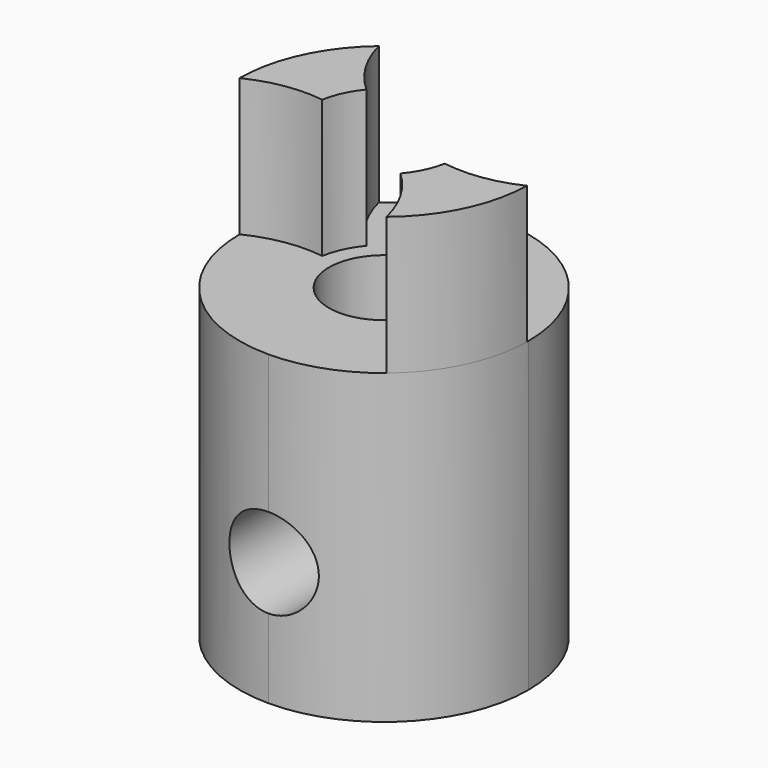
from build123d import *

# Parameters (mm, degrees)
F0_R        = 8.001
F0_R_2      = 3.048
F1_DEPTH    = 17.018
F3_W        = 16.002
F3_H        = 16.002
F4_DEPTH    = 17.018
F5_R        = 2.4765
F6_DEPTH    = 25.4
F7_T1_DEPTH = 57.023
F2_R        = 3.048
F8_DEPTH    = 25.4
F10_DEPTH   = 7.62
F11_SIZE    = 1.905


# Not quite as in the source:
# - a fillet or chamfer that OpenCascade refuses, or shapes differently, is made with other operations: its cross-section is extruded or revolved along the edge and cut away or added


with BuildPart() as f1:
    # F0 (on Top) → F1 (new body)
    with BuildSketch(Plane.XY):
        Circle(F0_R)
        Circle(F0_R_2, mode=Mode.SUBTRACT)
    extrude(amount=F1_DEPTH)

    # F3 (on Top) → F4 (join)
    with BuildSketch(Plane.XY):
        Rectangle(F3_W, F3_H)
    extrude(amount=F4_DEPTH)

    # F5 (on face) → F6 (cut)
    with BuildSketch(Plane.XZ.offset(8.001)):
        with Locations((0, 6.858)):
            Circle(F5_R)
    extrude(amount=-F6_DEPTH, mode=Mode.SUBTRACT)

    # F7: fillet of radius 8.001 on 4 edges, made by hand

    # F7_s2 → F7_t1 (cut)
    with BuildSketch(Plane.XY.offset(-20.0025)):
        with BuildLine():
            ThreePointArc((8.001, 0), (5.6575613563, -5.6575613563), (0, -8.001))
            Line((0, -8.001), (8.001, -8.001))
            Line((8.001, -8.001), (8.001, 0))
        make_face()
        with BuildLine():
            ThreePointArc((8.001, 0), (5.6575613563, 5.6575613563), (0, 8.001))
            Line((0, 8.001), (8.001, 8.001))
            Line((8.001, 8.001), (8.001, 0))
        make_face()
        with BuildLine():
            ThreePointArc((-8.001, 0), (-5.6575613563, -5.6575613563), (0, -8.001))
            Line((0, -8.001), (-8.001, -8.001))
            Line((-8.001, -8.001), (-8.001, 0))
        make_face()
        with BuildLine():
            ThreePointArc((0, 8.001), (-5.6575613563, 5.6575613563), (-8.001, 0))
            Line((-8.001, 0), (-8.001, 8.001))
            Line((-8.001, 8.001), (0, 8.001))
        make_face()
    extrude(amount=F7_T1_DEPTH, mode=Mode.SUBTRACT)

    # F2 (on face) → F8 (cut)
    with BuildSketch(Plane.XY.offset(17.018)):
        Circle(F2_R)
    extrude(amount=-F8_DEPTH, mode=Mode.SUBTRACT)

    # F9 (on face) → F10 (join)
    with BuildSketch(Plane.XY.offset(17.018)):
        with BuildLine():
            ThreePointArc((-3.0492599206, 2.589597302), (-4.3737921452, 4.1887242953), (-5.1697063492, 6.1065650953))
            ThreePointArc((-5.1697063492, 6.1065650953), (-7.2587471887, 3.3655), (-8.001, 0))
            ThreePointArc((-8.001, 0), (-6.0229894511, 0.6317175182), (-3.9466720244, 0.6540490669))
            ThreePointArc((-3.9466720244, 0.6540490669), (-3.6217185151, 1.6792007416), (-3.0492599206, 2.589597302))
        make_face()
        with BuildLine():
            ThreePointArc((3.0127388708, -2.6319963424), (4.3147732675, -4.2494941582), (5.0837832604, -6.1782804049))
            ThreePointArc((5.0837832604, -6.1782804049), (7.2109611489, -3.4667045316), (8.0002172314, -0.1119162637))
            ThreePointArc((8.0002172314, -0.1119162637), (6.0135638704, -0.7159039933), (3.9371372089, -0.7091902765))
            ThreePointArc((3.9371372089, -0.7091902765), (3.5978758903, -1.729696277), (3.0127388708, -2.6319963424))
        make_face()
    extrude(amount=F10_DEPTH)

    # F11
    f11_edges = [f1.edges().sort_by_distance(p)[0] for p in [
        (-3.048, 0, 0),
    ]]
    chamfer(f11_edges, length=F11_SIZE)


solid = f1.part
